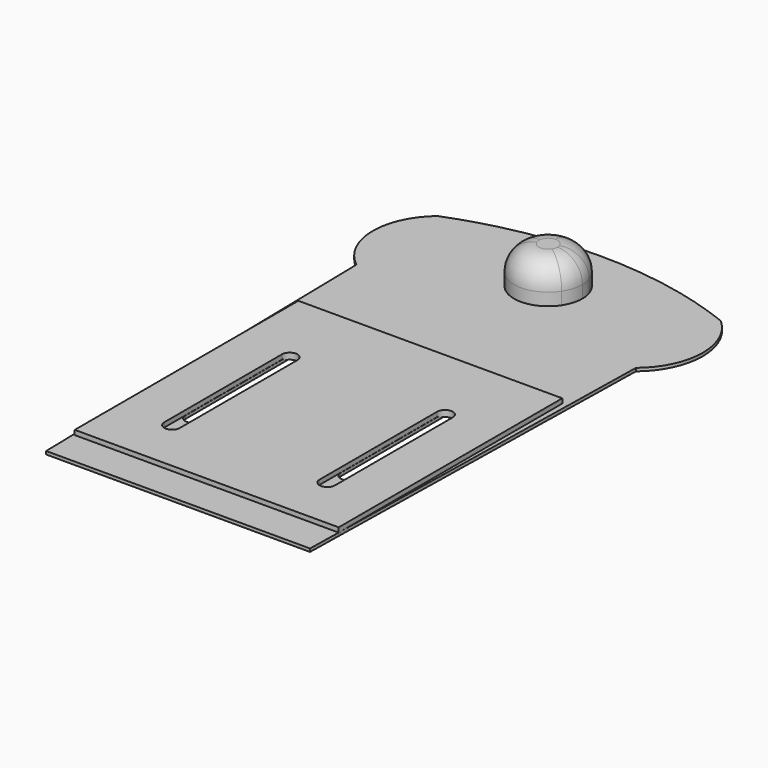
from build123d import *

# Parameters (mm, degrees)
F1_DEPTH = 12.5
F2_R     = 8
F3_W     = 85
F3_H     = 90
F4_DEPTH = 2
F5_DEPTH = 0.5


with BuildPart() as f1:
    # F0 (on Top) → F1 (new body)
    with BuildSketch(Plane.XY):
        with BuildLine():
            ThreePointArc((9.1898767867, 97.9546576073), (9.2825168111, 102.7916529277), (10.4312872179, 107.4911669936))
            ThreePointArc((10.4312872179, 107.4911669936), (6.4263972438, 112.9275650916), (0, 115))
            ThreePointArc((0, 115), (-7.2805617511, 112.2458123061), (-10.9152992151, 105.3624401069))
            ThreePointArc((-10.9152992151, 105.3624401069), (-10.3976417078, 102.6806649391), (-10.2241559556, 99.9549008188))
            ThreePointArc((-10.2241559556, 99.9549008188), (-10.2241569084, 99.9485001223), (-10.2241597667, 99.9420994264))
            ThreePointArc((-10.2241597667, 99.9420994264), (-1.1202305864, 93.0571903319), (9.1898767867, 97.9546576073))
        make_face()
        with BuildLine():
            ThreePointArc((11, 104), (10.8568908855, 105.768592746), (10.4312872179, 107.4911669936))
            ThreePointArc((10.4312872179, 107.4911669936), (9.2825168111, 102.7916529277), (9.1898767867, 97.9546576073))
            ThreePointArc((9.1898767867, 97.9546576073), (10.5377569875, 100.8447380976), (11, 104))
        make_face()
        with BuildLine():
            ThreePointArc((-10.2241559556, 99.9549008188), (-10.3976417078, 102.6806649391), (-10.9152992151, 105.3624401069))
            ThreePointArc((-10.9152992151, 105.3624401069), (-10.9116545392, 102.6086714205), (-10.2241597667, 99.9420994264))
            ThreePointArc((-10.2241597667, 99.9420994264), (-10.2241569084, 99.9485001223), (-10.2241559556, 99.9549008188))
        make_face()
    extrude(amount=F1_DEPTH)

    # F2
    f2_edges = [f1.edges().sort_by_distance(p)[0] for p in [
        (10.915299, 102.63756, 12.5),
    ]]
    fillet(f2_edges, radius=F2_R)

    # F0 (on Top) → F5 (join, symmetric)
    with BuildSketch(Plane.XY):
        with BuildLine():
            Line((45.0553547106, 83), (45.720910672, 116.3382926096))
            ThreePointArc((45.720910672, 116.3382926096), (37.1086608449, 119.3647656987), (28.2985051586, 121.7546492163))
            ThreePointArc((28.2985051586, 121.7546492163), (17.3640362052, 117.1292947522), (10.4312872179, 107.4911669936))
            ThreePointArc((10.4312872179, 107.4911669936), (10.8568908855, 105.768592746), (11, 104))
            ThreePointArc((11, 104), (10.5377569875, 100.8447380976), (9.1898767867, 97.9546576073))
            ThreePointArc((9.1898767867, 97.9546576073), (11.6452400122, 89.6864424383), (17.093512965, 83))
            Line((17.093512965, 83), (45.0553547106, 83))
        make_face()
        with BuildLine():
            ThreePointArc((53.0502116449, 99.9549008188), (51.1343756472, 108.9289492269), (45.720910672, 116.3382926096))
            Line((45.720910672, 116.3382926096), (45.0553547106, 83))
            ThreePointArc((45.0553547106, 83), (50.9512598026, 90.5822491239), (53.0502116449, 99.9549008188))
        make_face()
        with BuildLine():
            ThreePointArc((-29.8816593085, 121.3758066378), (-37.8142067265, 119.1431314413), (-45.5824041707, 116.3926304799))
            Line((-45.5824041707, 116.3926304799), (-44.9446452894, 83))
            Line((-44.9446452894, 83), (-18.5036666218, 83))
            ThreePointArc((-18.5036666218, 83), (-12.4074090251, 90.514917343), (-10.2241597667, 99.9420994264))
            ThreePointArc((-10.2241597667, 99.9420994264), (-10.9116545392, 102.6086714205), (-10.9152992151, 105.3624401069))
            ThreePointArc((-10.9152992151, 105.3624401069), (-17.8541188437, 116.3826843124), (-29.8816593085, 121.3758066378))
        make_face()
        with BuildLine():
            Line((-44.9446452894, 83), (-45.5824041707, 116.3926304799))
            ThreePointArc((-45.5824041707, 116.3926304799), (-53.2202358169, 99.5443516753), (-44.9446452894, 83))
        make_face()
        with BuildLine():
            ThreePointArc((10.4312872179, 107.4911669936), (17.3640362052, 117.1292947522), (28.2985051586, 121.7546492163))
            ThreePointArc((28.2985051586, 121.7546492163), (-0.8139254821, 124.9973500732), (-29.8816593085, 121.3758066378))
            ThreePointArc((-29.8816593085, 121.3758066378), (-17.8541188437, 116.3826843124), (-10.9152992151, 105.3624401069))
            ThreePointArc((-10.9152992151, 105.3624401069), (-7.2805617511, 112.2458123061), (0, 115))
            ThreePointArc((0, 115), (6.4263972438, 112.9275650916), (10.4312872179, 107.4911669936))
        make_face()
        with BuildLine():
            ThreePointArc((17.093512965, 83), (31.0744338378, 77.9791230117), (45.0553547106, 83))
            Line((45.0553547106, 83), (17.093512965, 83))
        make_face()
        with BuildLine():
            Line((42.797318697, -30.1070408914), (45.0553547106, 83))
            ThreePointArc((45.0553547106, 83), (31.0744338378, 77.9791230117), (17.093512965, 83))
            Line((17.093512965, 83), (-18.5036666218, 83))
            ThreePointArc((-18.5036666218, 83), (-31.7241559556, 78.4549008188), (-44.9446452894, 83))
            Line((-44.9446452894, 83), (-42.5, -45))
            Line((-42.5, -45), (42.5, -45))
            Line((42.5, -45), (42.7009939726, -34.9320323765))
            Line((42.7009939726, -34.9320323765), (-42.202681303, -34.9320323765))
            Line((-42.202681303, -34.9320323765), (-42.202681303, 55.0679676235))
            Line((-42.202681303, 55.0679676235), (42.797318697, 55.0679676235))
            Line((42.797318697, 55.0679676235), (42.797318697, -30.1070408914))
        make_face()
        with BuildLine():
            Line((-18.5036666218, 83), (-44.9446452894, 83))
            ThreePointArc((-44.9446452894, 83), (-31.7241559556, 78.4549008188), (-18.5036666218, 83))
        make_face()
        Polygon((42.7009939726, -34.9320323765), (42.797318697, -30.1070408914), (42.797318697, 55.0679676235), (-42.202681303, 55.0679676235), (-42.202681303, -34.9320323765), align=None)
        with BuildLine():
            ThreePointArc((-27.202681303, 39.3233826756), (-24.702681303, 41.8233826756), (-22.202681303, 39.3233826756))
            Line((-22.202681303, 39.3233826756), (-22.202681303, -8.0463153869))
            ThreePointArc((-22.202681303, -8.0463153869), (-24.702681303, -10.5463153869), (-27.202681303, -8.0463153869))
            Line((-27.202681303, -8.0463153869), (-27.202681303, 39.3233826756))
        make_face(mode=Mode.SUBTRACT)
        with BuildLine():
            Line((22.797318697, -8.0463153869), (22.797318697, 39.3233826756))
            ThreePointArc((22.797318697, 39.3233826756), (25.297318697, 41.8233826756), (27.797318697, 39.3233826756))
            Line((27.797318697, 39.3233826756), (27.797318697, -8.0463153869))
            ThreePointArc((27.797318697, -8.0463153869), (25.297318697, -10.5463153869), (22.797318697, -8.0463153869))
        make_face(mode=Mode.SUBTRACT)
        with BuildLine():
            Line((-18.5036666218, 83), (17.093512965, 83))
            ThreePointArc((17.093512965, 83), (11.6452400122, 89.6864424383), (9.1898767867, 97.9546576073))
            ThreePointArc((9.1898767867, 97.9546576073), (-1.1202305864, 93.0571903319), (-10.2241597667, 99.9420994264))
            ThreePointArc((-10.2241597667, 99.9420994264), (-12.4074090251, 90.514917343), (-18.5036666218, 83))
        make_face()
    extrude(amount=F5_DEPTH, both=True)


with BuildPart() as f4:
    # F3 (on face) → F4 (new body)
    with BuildSketch(Plane.XY):
        with Locations((0.2413462102, 11.2389419973)):
            Rectangle(F3_W, F3_H)
        with BuildLine():
            ThreePointArc((-27.2586537898, 30.8991409838), (-24.7586537898, 33.3991409838), (-22.2586537898, 30.8991409838))
            Line((-22.2586537898, 30.8991409838), (-22.2586537898, -16.4705570787))
            ThreePointArc((-22.2586537898, -16.4705570787), (-24.7586537898, -18.9705570787), (-27.2586537898, -16.4705570787))
            Line((-27.2586537898, -16.4705570787), (-27.2586537898, 30.8991409838))
        make_face(mode=Mode.SUBTRACT)
        with BuildLine():
            Line((22.7413462102, -16.4705570787), (22.7413462102, 30.8991409838))
            ThreePointArc((22.7413462102, 30.8991409838), (25.2413462102, 33.3991409838), (27.7413462102, 30.8991409838))
            Line((27.7413462102, 30.8991409838), (27.7413462102, -16.4705570787))
            ThreePointArc((27.7413462102, -16.4705570787), (25.2413462102, -18.9705570787), (22.7413462102, -16.4705570787))
        make_face(mode=Mode.SUBTRACT)
    extrude(amount=F4_DEPTH)


solid = Compound([f1.part, f4.part])
